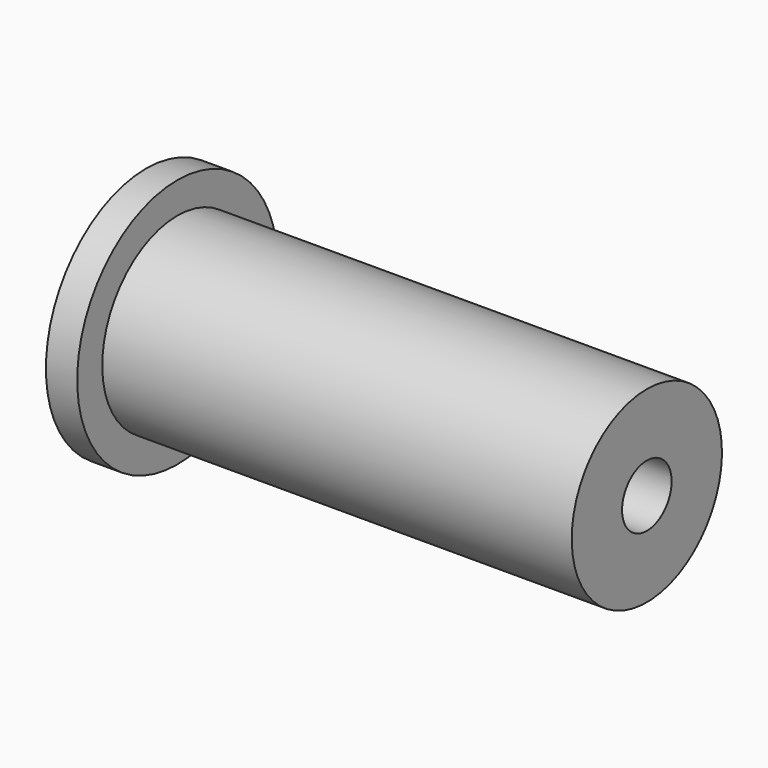
from build123d import *

# Parameters (mm, degrees)
F2_R     = 0.5
F3_DEPTH = 4.001


# Not quite as in the source:
# - a feature names something its author has since deleted; it is built from what else it names


with BuildPart() as f1:
    # F0 (on Front) → F1 (revolve)
    with BuildSketch(Plane.XZ):
        Polygon((0, 4), (0, 0.99), (16, 0.99), (16, 3), (1, 3), (1, 4), align=None)
    revolve(axis=Axis((-1.1582460975, 0, 0), (1, 0, 0)))

    # F2 (on Top) → F3 (cut, through all)
    with BuildSketch(Plane.XY):
        with Locations((2.5, 0)):
            Circle(F2_R)
        with Locations((13.275148347, 0)):
            Circle(F2_R)
    extrude(amount=-F3_DEPTH, mode=Mode.SUBTRACT)


solid = f1.part
